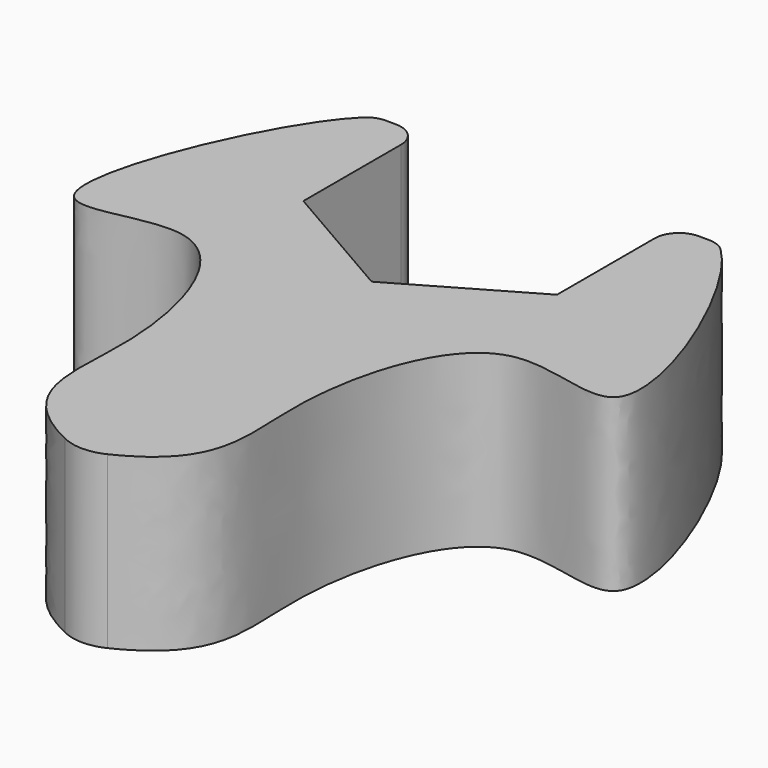
from build123d import *

# Parameters (mm, degrees)
F1_DEPTH = 7
F2_R     = 1
F4_R     = 2


with BuildPart() as f1:
    # F0 (on Top) → F1 (new body)
    with BuildSketch(Plane.XY):
        with BuildLine():
            Line((7, 3.0022213998), (5.2, 3.0022213998))
            Line((5.2, 3.0022213998), (5.2, -3.0022213998))
            Line((5.2, -3.0022213998), (0, -6.0044427996))
            Line((0, -6.0044427996), (0, -21.0044427996))
            add(Edge.make_bspline(
                [(7, 3.0022213998), (9.0188791452, 1.5366041561), (14.1530994004, -10.3624473952), (5.3831616493, -5.0907205572), (2.5568231001, -14.7335644159), (4.4003581826, -19.3230181565), (0, -21.0044427996)],
                knots=[0.1088687327, 0.1088687327, 0.1088687327, 0.1088687327, 0.3789912854, 0.5511278659, 0.7740225577, 1, 1, 1, 1], degree=3))
        make_face()
    extrude(amount=F1_DEPTH)

    # F2
    f2_edges = [f1.edges().sort_by_distance(p)[0] for p in [
        (5.2, 3.002221, 3.5),
        (7, 3.002221, 3.5),
    ]]
    fillet(f2_edges, radius=F2_R)

    # F3: F1 across plane


with BuildPart() as f1_1:
    add(f1.part)
    add(f1.part.mirror(Plane.YZ))

    # F4
    f4_edges = [f1_1.edges().sort_by_distance(p)[0] for p in [
        (0, -21.004443, 3.5),
    ]]
    fillet(f4_edges, radius=F4_R)


solid = f1_1.part
